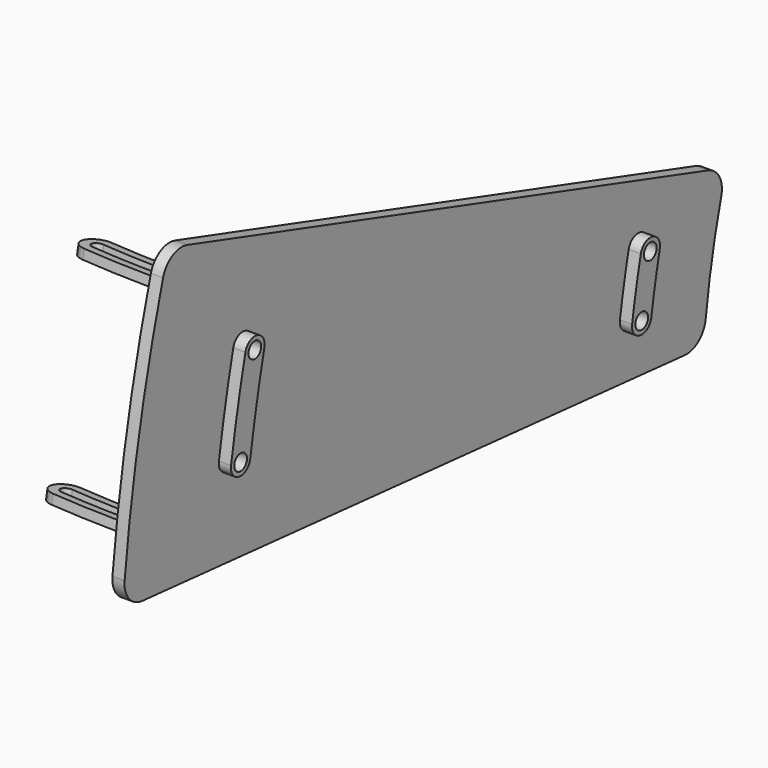
from build123d import *

# Parameters (mm, degrees)
F1_DEPTH  = 12.7
F2_DEPTH  = 12.7
F4_D      = 16.66748
F7_DEPTH  = 25.4
F10_DEPTH = 9.652
F13_D     = 16.66748
F15_D     = 16.66748


# Not quite as in the source:
# - a feature of the source that left no trace in its solid (it failed there, or was rolled back) is left out
# - a pattern or mirror of a feature is missing from the dataset's text; its kind, count and spacing are read off the source's solid


with BuildPart() as f1:
    # F0 (on Right) → F1 (new body)
    with BuildSketch(Plane.YZ):
        with BuildLine():
            ThreePointArc((-756.3314490517, 92.7725130381), (-747.9999137871, 145.3964544769), (-736.0115033336, 197.3095713861))
            ThreePointArc((-736.0115033336, 197.3095713861), (-738.3291312366, 216.1993713631), (-753.1189788115, 228.1766979004))
            Line((-753.1189788115, 228.1766979004), (-1433.4591504296, 436.1775621929))
            ThreePointArc((-1433.4591504296, 436.1775621929), (-1453.0143855451, 434.2043994356), (-1465.30717803, 418.8685641269))
            ThreePointArc((-1465.30717803, 418.8685641269), (-1495.9998275742, 290.7929089539), (-1515.5200833468, 160.5455604257))
            ThreePointArc((-1515.5200833468, 160.5455604257), (-1509.8673096495, 141.7214604148), (-1492.4751711568, 132.5664557537))
            Line((-1492.4751711568, 132.5664557537), (-783.7562532192, 70.5615848078))
            ThreePointArc((-783.7562532192, 70.5615848078), (-765.5565598439, 76.1263941769), (-756.3314490517, 92.7725130381))
        make_face()
        with BuildLine():
            ThreePointArc((-868.3901696878, 137.4879790683), (-863.196533516, 167.7279226013), (-856.9770599652, 197.7736575783))
            ThreePointArc((-856.9770599652, 197.7736575783), (-841.8007632153, 207.3788653824), (-832.1955554113, 192.2025686325))
            ThreePointArc((-832.1955554113, 192.2025686325), (-838.239832524, 163.0031923871), (-843.2871690853, 133.6150782495))
            ThreePointArc((-843.2871690853, 133.6150782495), (-857.775119796, 123.0000283577), (-868.3901696878, 137.4879790683))
        make_face(mode=Mode.SUBTRACT)
        with BuildLine():
            ThreePointArc((-1392.344253737, 220.5256653672), (-1383.7998405062, 268.9834407823), (-1373.5694803277, 317.1135013085))
            ThreePointArc((-1373.5694803277, 317.1135013085), (-1358.3381021148, 326.6311227412), (-1348.8204806822, 311.3997445282))
            ThreePointArc((-1348.8204806822, 311.3997445282), (-1358.8665100466, 264.1368922998), (-1367.2569698858, 216.5522299552))
            ThreePointArc((-1367.2569698858, 216.5522299552), (-1381.7873295174, 205.9953057356), (-1392.344253737, 220.5256653672))
        make_face(mode=Mode.SUBTRACT)
        with BuildLine():
            ThreePointArc((-1348.8204806822, 311.3997445282), (-1358.3381021148, 326.6311227412), (-1373.5694803277, 317.1135013085))
            ThreePointArc((-1373.5694803277, 317.1135013085), (-1383.7998405062, 268.9834407823), (-1392.344253737, 220.5256653672))
            ThreePointArc((-1392.344253737, 220.5256653672), (-1381.7873295174, 205.9953057356), (-1367.2569698858, 216.5522299552))
            ThreePointArc((-1367.2569698858, 216.5522299552), (-1358.8665100466, 264.1368922998), (-1348.8204806822, 311.3997445282))
        make_face()
        with BuildLine():
            ThreePointArc((-832.1955554113, 192.2025686325), (-841.8007632153, 207.3788653824), (-856.9770599652, 197.7736575783))
            ThreePointArc((-856.9770599652, 197.7736575783), (-863.196533516, 167.7279226013), (-868.3901696878, 137.4879790683))
            ThreePointArc((-868.3901696878, 137.4879790683), (-857.775119796, 123.0000283577), (-843.2871690853, 133.6150782495))
            ThreePointArc((-843.2871690853, 133.6150782495), (-838.239832524, 163.0031923871), (-832.1955554113, 192.2025686325))
        make_face()
    extrude(amount=-F1_DEPTH)

    # F4 (through all)
    with Locations(Plane.YZ.offset(12.7)):
        with Locations((-1361.194980505, 314.2566229184), (-1379.8006118114, 218.5389476612), (-844.5863076883, 194.9881131054), (-855.8386693866, 135.5515286589)):
            Hole(F4_D / 2)

    # F6 (on face) → F7 (join, symmetric)
    with BuildSketch(Plane(origin=(0, 0, 0), x_dir=(1, 0, 0), z_dir=(0, -0.1908089954, -0.9816271834))):
        with BuildLine():
            ThreePointArc((-38.1, 829.9252514334), (-33.6098719395, 828.0653794939), (-31.75, 823.5752514334))
            ThreePointArc((-31.75, 823.5752514334), (-33.6098719395, 819.0851233729), (-38.1, 817.2252514334))
            Line((-38.1, 817.2252514334), (-38.1, 810.8752514334))
            ThreePointArc((-38.1, 810.8752514334), (-29.1197438789, 814.5949953123), (-25.4, 823.5752514334))
            ThreePointArc((-25.4, 823.5752514334), (-29.1197438789, 832.5555075545), (-38.1, 836.2752514334))
            Line((-38.1, 836.2752514334), (-38.1, 829.9252514334))
        make_face()
        with BuildLine():
            ThreePointArc((-38.1, 817.2252514334), (-44.45, 823.5752514334), (-38.1, 829.9252514334))
            Line((-38.1, 829.9252514334), (-38.1, 836.2752514334))
            ThreePointArc((-38.1, 836.2752514334), (-50.8, 823.5752514334), (-38.1, 810.8752514334))
            Line((-38.1, 810.8752514334), (-38.1, 817.2252514334))
        make_face()
        with BuildLine():
            Line((-12.7, 836.2752514334), (-38.1, 836.2752514334))
            ThreePointArc((-38.1, 836.2752514334), (-29.1197438789, 832.5555075545), (-25.4, 823.5752514334))
            ThreePointArc((-25.4, 823.5752514334), (-29.1197438789, 814.5949953123), (-38.1, 810.8752514334))
            Line((-38.1, 810.8752514334), (-12.7, 810.8752514334))
            Line((-12.7, 810.8752514334), (-12.7, 836.2752514334))
        make_face()
    extrude(amount=F7_DEPTH, both=True)


with BuildPart() as f2:
    # F0 (on Right) → F2 (new body)
    with BuildSketch(Plane.YZ):
        with BuildLine():
            ThreePointArc((-1348.8204806822, 311.3997445282), (-1358.3381021148, 326.6311227412), (-1373.5694803277, 317.1135013085))
            ThreePointArc((-1373.5694803277, 317.1135013085), (-1383.7998405062, 268.9834407823), (-1392.344253737, 220.5256653672))
            ThreePointArc((-1392.344253737, 220.5256653672), (-1381.7873295174, 205.9953057356), (-1367.2569698858, 216.5522299552))
            ThreePointArc((-1367.2569698858, 216.5522299552), (-1358.8665100466, 264.1368922998), (-1348.8204806822, 311.3997445282))
        make_face()
    extrude(amount=F2_DEPTH)

    # F15 (through all)
    with Locations(Plane.YZ.offset(12.7)):
        with Locations((-1361.194980505, 314.2566229184), (-1379.8006118114, 218.5389476612)):
            Hole(F15_D / 2)


with BuildPart() as f2b:
    # F0 (on Right) → F2, piece 2 (new body)
    with BuildSketch(Plane.YZ):
        with BuildLine():
            ThreePointArc((-832.1955554113, 192.2025686325), (-841.8007632153, 207.3788653824), (-856.9770599652, 197.7736575783))
            ThreePointArc((-856.9770599652, 197.7736575783), (-863.196533516, 167.7279226013), (-868.3901696878, 137.4879790683))
            ThreePointArc((-868.3901696878, 137.4879790683), (-857.775119796, 123.0000283577), (-843.2871690853, 133.6150782495))
            ThreePointArc((-843.2871690853, 133.6150782495), (-838.239832524, 163.0031923871), (-832.1955554113, 192.2025686325))
        make_face()
    extrude(amount=F2_DEPTH)

    # F13 (through all)
    with Locations(Plane.YZ.offset(12.7)):
        with Locations((-844.5863076883, 194.9881131054), (-855.8386693866, 135.5515286589)):
            Hole(F13_D / 2)


with BuildPart() as f10:
    # F9 (on face) → F10 (new body)
    with BuildSketch(Plane(origin=(0, -19.3861939303, -99.7333218383), x_dir=(1, 0, 0), z_dir=(0, -0.1908089954, -0.9816271834))):
        with BuildLine():
            Line((-12.7, 1458.0670480707), (-12.7, 1474.0815496381))
            ThreePointArc((-12.7, 1474.0815496381), (-65.1564294406, 1474.0147594815), (-117.4371862954, 1469.7247812442))
            ThreePointArc((-117.4371862954, 1469.7247812442), (-131.3697565808, 1451.8919044925), (-113.5368798291, 1437.9593342071))
            ThreePointArc((-113.5368798291, 1437.9593342071), (-63.2019841466, 1442.064066527), (-12.7, 1442.0518993386))
            Line((-12.7, 1442.0518993386), (-12.7, 1458.0670480707))
        make_face()
        with BuildLine():
            ThreePointArc((-38.1, 1464.9252514334), (-31.75, 1458.5752514334), (-38.1, 1452.2252514334))
            ThreePointArc((-38.1, 1452.2252514334), (-76.4781643786, 1451.0526924613), (-114.7131627316, 1447.5393896627))
            ThreePointArc((-114.7131627316, 1447.5393896627), (-121.7897011252, 1453.068187395), (-116.2609033929, 1460.1447257886))
            ThreePointArc((-116.2609033929, 1460.1447257886), (-77.2534808307, 1463.7290044013), (-38.1, 1464.9252514334))
        make_face(mode=Mode.SUBTRACT)
    extrude(amount=F10_DEPTH)


with BuildPart() as f10_copies_1:
    # F10_copies: instance of F10
    add(f10.part.mirror(Plane(origin=(0, 0, 0), x_dir=(0, 0.9816271834, -0.1908089954), z_dir=(0, 0.1908089954, 0.9816271834))))


solid = Compound([f1.part, f2.part, f2b.part, f10.part, f10_copies_1.part])
